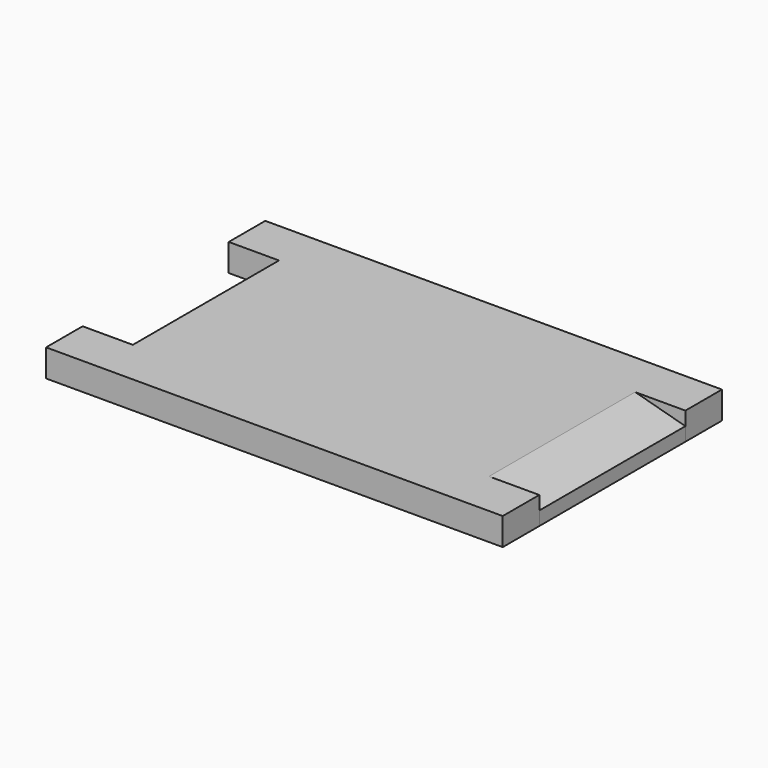
from build123d import *

# Parameters (mm, degrees)
F2_DEPTH      = 30
F0_W          = 55
F0_H          = 200
F3_DEPTH      = 30
F4_DEPTH      = 150.001
F4_DEPTH_BACK = 150.001


# Not quite as in the source:
# - a feature of the source that left no trace in its solid (it failed there, or was rolled back) is left out


with BuildPart() as f2:
    # F0 (on Top) → F2 (new body)
    with BuildSketch(Plane.XY):
        Polygon((250, 150), (-250, 150), (-250, 100), (-195, 100), (-195, -100), (-250, -100), (-250, -150), (250, -150), (250, -100), (195, -100), (195, 100), (250, 100), align=None)
    extrude(amount=-F2_DEPTH)


with BuildPart() as f3:
    # F0 (on Top) → F3 (new body, through all)
    with BuildSketch(Plane.XY):
        with Locations((222.5, 0)):
            Rectangle(F0_W, F0_H)
    extrude(amount=-F3_DEPTH)

    # F1 (on Front) → F4 (cut, two sides)
    with BuildSketch(Plane.XZ) as f4_sk:
        Polygon((250, -15), (250, 0), (195, 0), align=None)
    extrude(amount=-F4_DEPTH, mode=Mode.SUBTRACT)
    extrude(f4_sk.sketch, amount=F4_DEPTH_BACK, mode=Mode.SUBTRACT)


solid = Compound([f2.part, f3.part])
